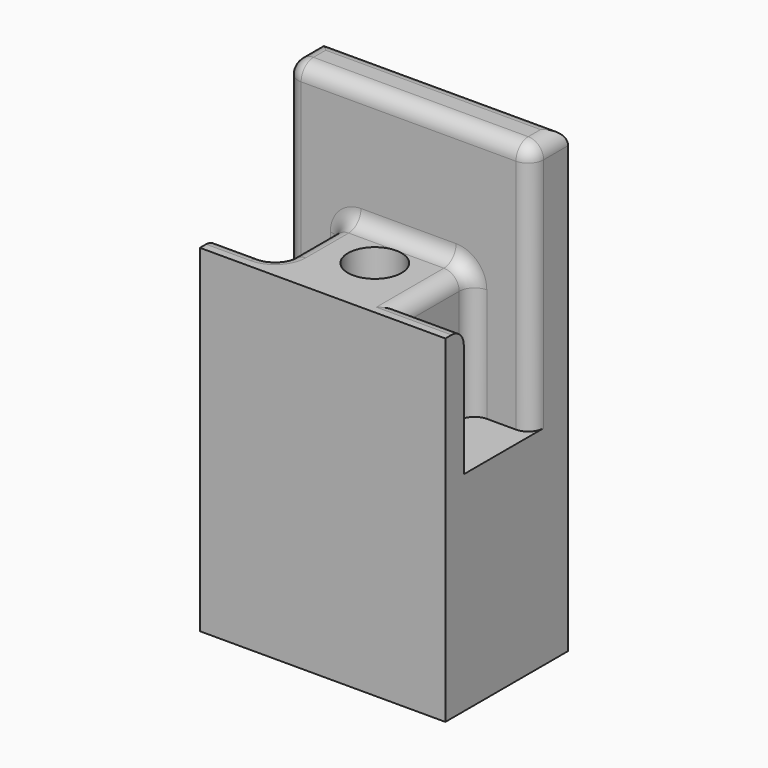
from build123d import *

# Parameters (mm, degrees)
F0_W     = 16
F0_H     = 10
F1_DEPTH = 30
F2_W     = 16
F2_H     = 7
F3_DEPTH = 8
F4_W     = 3.9
F4_H     = 5.5
F5_DEPTH = 8.4
F6_R     = 1.75
F7_DEPTH = 5
F8_F1_R  = 1
F8_F2_R  = 1
F8_F3_R  = 0.9999


# Not quite as in the source:
# - a fillet or chamfer is up to 0.001 mm smaller than in the source, because OpenCascade refuses the exact size
# - a feature names something its author has since deleted; it is built from what else it names


with BuildPart() as f1:
    # F0 (on Top) → F1 (new body)
    with BuildSketch(Plane.XY):
        Rectangle(F0_W, F0_H)
    extrude(amount=F1_DEPTH)

    # F2 (on face) → F3 (cut)
    with BuildSketch(Plane.XY.offset(30)):
        with Locations((0, -1.5)):
            Rectangle(F2_W, F2_H)
    extrude(amount=-F3_DEPTH, mode=Mode.SUBTRACT)

    # F4 (on face) → F5 (cut)
    with BuildSketch(Plane.XY.offset(22)):
        with Locations((-6.05, -0.75)):
            Rectangle(F4_W, F4_H)
        with Locations((6.05, -0.75)):
            Rectangle(F4_W, F4_H)
    extrude(amount=-F5_DEPTH, mode=Mode.SUBTRACT)

    # F6 (on face) → F7 (cut)
    with BuildSketch(Plane.XY.offset(22)):
        with Locations((0, -0.75)):
            Circle(F6_R)
    extrude(amount=-F7_DEPTH, mode=Mode.SUBTRACT)

    # F8: fillet of radius 1 on 13 edges, made by hand

    # F8_f1
    f8_f1_edges = [f1.edges().sort_by_distance(p)[0] for p in [
        (-4.1, -3.5, 17.8),
    ]]
    fillet(f8_f1_edges, radius=F8_F1_R)

    # F8_f2
    f8_f2_edges = [f1.edges().sort_by_distance(p)[0] for p in [
        (4.1, -0.75, 22),
        (-4.1, -0.25, 22),
        (6.05, -3.5, 22),
        (8, 3.5, 30),
        (-8, 3.5, 30),
        (0, 2, 30),
        (0, 5, 30),
        (-8, 2, 21.8),
        (8, 2, 21.8),
        (-4.3928932188, -3.2071067812, 22),
    ]]
    fillet(f8_f2_edges, radius=F8_F2_R)

    # F8_f3 (radius 1 in the source; OpenCascade refuses exactly that, so slightly less here)
    f8_f3_edges = [f1.edges().sort_by_distance(p)[0] for p in [
        (4.1, 2, 17.3),
        (-4.1, 2, 17.3),
        (0, 2, 22),
        (3.8071067812, 2, 21.7071067812),
        (-3.8071067812, 2, 21.7071067812),
    ]]
    fillet(f8_f3_edges, radius=F8_F3_R)


solid = f1.part
